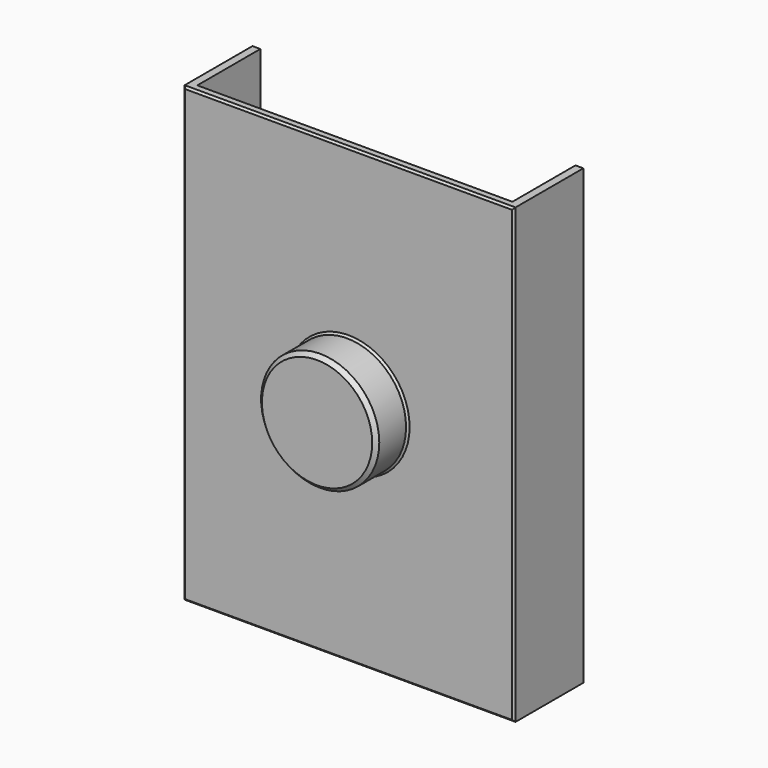
from build123d import *

# Parameters (mm, degrees)
F0_W     = 2
F0_H     = 115
F1_DEPTH = 20
F2_DEPTH = 20
F0_W_2   = 80
F0_R     = 15
F3_DEPTH = 2
F0_R_2   = 13
F4_DEPTH = 12
F5_DEPTH = 10
F6_SIZE  = 0.5
F7_SIZE  = 1


with BuildPart() as f1:
    # F0 (on Front) → F1 (new body)
    with BuildSketch(Plane.XZ):
        with Locations((-41, 0)):
            Rectangle(F0_W, F0_H)
    extrude(amount=-F1_DEPTH)



with BuildPart() as f2:
    # F0 (on Front) → F2 (new body)
    with BuildSketch(Plane.XZ):
        with Locations((41, 0)):
            Rectangle(F0_W, F0_H)
    extrude(amount=-F2_DEPTH)


with BuildPart() as f1_1:
    add(f1.part)

    add(f2.part)  # F3 merges F2
    # F0 (on Front) → F3 (join)
    with BuildSketch(Plane.XZ):
        Rectangle(F0_W_2, F0_H)
        Circle(F0_R, mode=Mode.SUBTRACT)
        with Locations((41, 0)):
            Rectangle(F0_W, F0_H)
        with Locations((-41, 0)):
            Rectangle(F0_W, F0_H)
    extrude(amount=F3_DEPTH)

    # F0 (on Front) → F4 (join)
    with BuildSketch(Plane.XZ):
        Circle(F0_R)
        Circle(F0_R_2, mode=Mode.SUBTRACT)
        Circle(F0_R_2)
    extrude(amount=F4_DEPTH)

    # F0 (on Front) → F5 (cut)
    with BuildSketch(Plane.XZ):
        Circle(F0_R_2)
    extrude(amount=F5_DEPTH, mode=Mode.SUBTRACT)

    # F6
    f6_edges = [f1_1.edges().sort_by_distance(p)[0] for p in [
        (42, -2, 0),
        (0, -2, 57.5),
        (-42, -2, 0),
        (0, -2, -57.5),
        (-15, -2, 0),
    ]]
    chamfer(f6_edges, length=F6_SIZE)

    # F7
    f7_edges = [f1_1.edges().sort_by_distance(p)[0] for p in [
        (-15, -12, 0),
    ]]
    chamfer(f7_edges, length=F7_SIZE)


solid = f1_1.part
